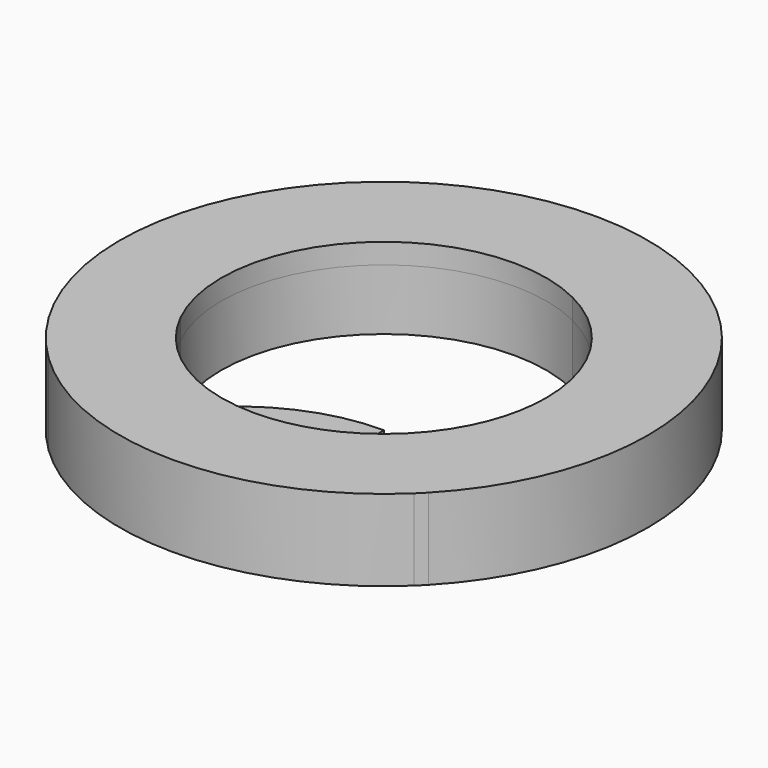
from build123d import *

# Parameters (mm, degrees)
F1_DEPTH = 20
F2_DEPTH = 15
F3_DEPTH = 15
F4_DEPTH = 5
F5_R     = 5


# Not quite as in the source:
# - a feature names something its author has since deleted; it is built from what else it names


with BuildPart() as f1:
    # F0 (on Top) → F1 (new body)
    with BuildSketch(Plane.XY):
        with BuildLine():
            ThreePointArc((-41.5739709642, -27.7777777778), (-35.3553390593, 35.3553390593), (27.7777777778, 41.5739709642))
            ThreePointArc((27.7777777778, 41.5739709642), (37.1759673359, 44.3146083461), (46.9444444444, 44.9579707705))
            ThreePointArc((46.9444444444, 44.9579707705), (-45.9619407771, 45.9619407771), (-44.9579707705, -46.9444444444))
            ThreePointArc((-44.9579707705, -46.9444444444), (-44.9806919732, -43.6819144147), (-44.7669675939, -40.426313036))
            ThreePointArc((-44.7669675939, -40.426313036), (-43.6312477339, -33.9857264796), (-41.5739709642, -27.7777777778))
        make_face()
        with BuildLine():
            ThreePointArc((45, -45), (36.220156419, -44.1351826403), (27.7777777778, -41.5739709642))
            ThreePointArc((27.7777777778, -41.5739709642), (14.5138115564, -47.8471448898), (0, -50))
            ThreePointArc((0, -50), (-12.7926961833, -48.3357727192), (-24.7337942073, -43.4538769745))
            ThreePointArc((-24.7337942073, -43.4538769745), (-29.4930498897, -42.6445374906), (-33.6593211472, -45.0833340912))
            ThreePointArc((-33.6593211472, -45.0833340912), (-40.9388886222, -46.870964929), (-44.7669675939, -40.426313036))
            ThreePointArc((-44.7669675939, -40.426313036), (-44.9806919732, -43.6819144147), (-44.9579707705, -46.9444444444))
            ThreePointArc((-44.9579707705, -46.9444444444), (0, -65), (44.9579707705, -46.9444444444))
            ThreePointArc((44.9579707705, -46.9444444444), (44.9894914656, -45.9724493115), (45, -45))
        make_face()
        with BuildLine():
            ThreePointArc((27.7777777778, 41.5739709642), (44.0958551844, 23.5702260396), (50, 0))
            ThreePointArc((50, 0), (47.8471448898, -14.5138115564), (41.5739709642, -27.7777777778))
            ThreePointArc((41.5739709642, -27.7777777778), (44.1351826403, -36.220156419), (45, -45))
            ThreePointArc((45, -45), (45.9724493115, -44.9894914656), (46.9444444444, -44.9579707705))
            ThreePointArc((46.9444444444, -44.9579707705), (60.317447264, -24.2240697562), (65, 0))
            ThreePointArc((65, 0), (60.317447264, 24.2240697562), (46.9444444444, 44.9579707705))
            ThreePointArc((46.9444444444, 44.9579707705), (37.1759673359, 44.3146083461), (27.7777777778, 41.5739709642))
        make_face()
        with BuildLine():
            ThreePointArc((45, -45), (44.1351826403, -36.220156419), (41.5739709642, -27.7777777778))
            ThreePointArc((41.5739709642, -27.7777777778), (35.3553390593, -35.3553390593), (27.7777777778, -41.5739709642))
            ThreePointArc((27.7777777778, -41.5739709642), (36.220156419, -44.1351826403), (45, -45))
        make_face()
        with BuildLine():
            ThreePointArc((46.9444444444, -44.9579707705), (45.9724493115, -44.9894914656), (45, -45))
            ThreePointArc((45, -45), (44.9894914656, -45.9724493115), (44.9579707705, -46.9444444444))
            ThreePointArc((44.9579707705, -46.9444444444), (45.9619407771, -45.9619407771), (46.9444444444, -44.9579707705))
        make_face()
        with BuildLine():
            ThreePointArc((-35.8322566591, -17.7777777778), (-28.2842712475, 28.2842712475), (17.7777777778, 35.8322566591))
            ThreePointArc((17.7777777778, 35.8322566591), (22.5931041578, 39.0247487976), (27.7777777778, 41.5739709642))
            ThreePointArc((27.7777777778, 41.5739709642), (-35.3553390593, 35.3553390593), (-41.5739709642, -27.7777777778))
            ThreePointArc((-41.5739709642, -27.7777777778), (-39.0247487976, -22.5931041578), (-35.8322566591, -17.7777777778))
        make_face()
        with BuildLine():
            ThreePointArc((17.7777777778, 35.8322566591), (33.993463424, 21.0818510678), (40, 0))
            Line((40, 0), (50, 0))
            ThreePointArc((50, 0), (44.0958551844, 23.5702260396), (27.7777777778, 41.5739709642))
            ThreePointArc((27.7777777778, 41.5739709642), (22.5931041578, 39.0247487976), (17.7777777778, 35.8322566591))
        make_face()
        with BuildLine():
            Line((50, 0), (40, 0))
            ThreePointArc((40, 0), (38.9441283531, -9.1298886531), (35.8322566591, -17.7777777778))
            ThreePointArc((35.8322566591, -17.7777777778), (39.0247487976, -22.5931041578), (41.5739709642, -27.7777777778))
            ThreePointArc((41.5739709642, -27.7777777778), (47.8471448898, -14.5138115564), (50, 0))
        make_face()
        with BuildLine():
            ThreePointArc((41.5739709642, -27.7777777778), (39.0247487976, -22.5931041578), (35.8322566591, -17.7777777778))
            ThreePointArc((35.8322566591, -17.7777777778), (28.2842712475, -28.2842712475), (17.7777777778, -35.8322566591))
            ThreePointArc((17.7777777778, -35.8322566591), (22.5931041578, -39.0247487976), (27.7777777778, -41.5739709642))
            ThreePointArc((27.7777777778, -41.5739709642), (35.3553390593, -35.3553390593), (41.5739709642, -27.7777777778))
        make_face()
        with BuildLine():
            ThreePointArc((27.7777777778, -41.5739709642), (22.5931041578, -39.0247487976), (17.7777777778, -35.8322566591))
            ThreePointArc((17.7777777778, -35.8322566591), (9.1298886531, -38.9441283531), (0, -40))
            Line((0, -40), (0, -50))
            ThreePointArc((0, -50), (14.5138115564, -47.8471448898), (27.7777777778, -41.5739709642))
        make_face()
        with BuildLine():
            ThreePointArc((0, -40), (-21.0818510678, -33.993463424), (-35.8322566591, -17.7777777778))
            ThreePointArc((-35.8322566591, -17.7777777778), (-39.0247487976, -22.5931041578), (-41.5739709642, -27.7777777778))
            ThreePointArc((-41.5739709642, -27.7777777778), (-38.1355654332, -32.3369548518), (-34.1997389873, -36.4743451373))
            ThreePointArc((-34.1997389873, -36.4743451373), (-29.6726945164, -40.2433994605), (-24.7337942073, -43.4538769745))
            ThreePointArc((-24.7337942073, -43.4538769745), (-12.7926961833, -48.3357727192), (0, -50))
            Line((0, -50), (0, -40))
        make_face()
        with BuildLine():
            ThreePointArc((-34.1997389873, -36.4743451373), (-38.1355654332, -32.3369548518), (-41.5739709642, -27.7777777778))
            ThreePointArc((-41.5739709642, -27.7777777778), (-43.6312477339, -33.9857264796), (-44.7669675939, -40.426313036))
            ThreePointArc((-44.7669675939, -40.426313036), (-40.7099854287, -35.1704182799), (-34.1997389873, -36.4743451373))
        make_face()
        with BuildLine():
            ThreePointArc((-32.2106591377, -41.0660656442), (-32.729295856, -38.564049664), (-34.1997389873, -36.4743451373))
            ThreePointArc((-34.1997389873, -36.4743451373), (-40.7099854287, -35.1704182799), (-44.7669675939, -40.426313036))
            ThreePointArc((-44.7669675939, -40.426313036), (-40.9388886222, -46.870964929), (-33.6593211472, -45.0833340912))
            ThreePointArc((-33.6593211472, -45.0833340912), (-32.5838900439, -43.2013096228), (-32.2106591377, -41.0660656442))
        make_face()
        with BuildLine():
            ThreePointArc((-24.7337942073, -43.4538769745), (-29.6726945164, -40.2433994605), (-34.1997389873, -36.4743451373))
            ThreePointArc((-34.1997389873, -36.4743451373), (-32.729295856, -38.564049664), (-32.2106591377, -41.0660656442))
            ThreePointArc((-32.2106591377, -41.0660656442), (-32.5838900439, -43.2013096228), (-33.6593211472, -45.0833340912))
            ThreePointArc((-33.6593211472, -45.0833340912), (-29.4930498897, -42.6445374906), (-24.7337942073, -43.4538769745))
        make_face()
    extrude(amount=F1_DEPTH)

    # F0 (on Top) → F2 (cut)
    with BuildSketch(Plane.XY):
        with BuildLine():
            ThreePointArc((17.7777777778, 35.8322566591), (33.993463424, 21.0818510678), (40, 0))
            Line((40, 0), (50, 0))
            ThreePointArc((50, 0), (44.0958551844, 23.5702260396), (27.7777777778, 41.5739709642))
            ThreePointArc((27.7777777778, 41.5739709642), (22.5931041578, 39.0247487976), (17.7777777778, 35.8322566591))
        make_face()
        with BuildLine():
            Line((50, 0), (40, 0))
            ThreePointArc((40, 0), (38.9441283531, -9.1298886531), (35.8322566591, -17.7777777778))
            ThreePointArc((35.8322566591, -17.7777777778), (39.0247487976, -22.5931041578), (41.5739709642, -27.7777777778))
            ThreePointArc((41.5739709642, -27.7777777778), (47.8471448898, -14.5138115564), (50, 0))
        make_face()
        with BuildLine():
            ThreePointArc((41.5739709642, -27.7777777778), (39.0247487976, -22.5931041578), (35.8322566591, -17.7777777778))
            ThreePointArc((35.8322566591, -17.7777777778), (28.2842712475, -28.2842712475), (17.7777777778, -35.8322566591))
            ThreePointArc((17.7777777778, -35.8322566591), (22.5931041578, -39.0247487976), (27.7777777778, -41.5739709642))
            ThreePointArc((27.7777777778, -41.5739709642), (35.3553390593, -35.3553390593), (41.5739709642, -27.7777777778))
        make_face()
        with BuildLine():
            ThreePointArc((27.7777777778, -41.5739709642), (22.5931041578, -39.0247487976), (17.7777777778, -35.8322566591))
            ThreePointArc((17.7777777778, -35.8322566591), (9.1298886531, -38.9441283531), (0, -40))
            Line((0, -40), (0, -50))
            ThreePointArc((0, -50), (14.5138115564, -47.8471448898), (27.7777777778, -41.5739709642))
        make_face()
        with BuildLine():
            ThreePointArc((0, -40), (-21.0818510678, -33.993463424), (-35.8322566591, -17.7777777778))
            ThreePointArc((-35.8322566591, -17.7777777778), (-39.0247487976, -22.5931041578), (-41.5739709642, -27.7777777778))
            ThreePointArc((-41.5739709642, -27.7777777778), (-38.1355654332, -32.3369548518), (-34.1997389873, -36.4743451373))
            ThreePointArc((-34.1997389873, -36.4743451373), (-29.6726945164, -40.2433994605), (-24.7337942073, -43.4538769745))
            ThreePointArc((-24.7337942073, -43.4538769745), (-12.7926961833, -48.3357727192), (0, -50))
            Line((0, -50), (0, -40))
        make_face()
        with BuildLine():
            ThreePointArc((-35.8322566591, -17.7777777778), (-28.2842712475, 28.2842712475), (17.7777777778, 35.8322566591))
            ThreePointArc((17.7777777778, 35.8322566591), (22.5931041578, 39.0247487976), (27.7777777778, 41.5739709642))
            ThreePointArc((27.7777777778, 41.5739709642), (-35.3553390593, 35.3553390593), (-41.5739709642, -27.7777777778))
            ThreePointArc((-41.5739709642, -27.7777777778), (-39.0247487976, -22.5931041578), (-35.8322566591, -17.7777777778))
        make_face()
    extrude(amount=F2_DEPTH, mode=Mode.SUBTRACT)


with BuildPart() as f3:
    # F0 (on Top) → F3 (new body)
    with BuildSketch(Plane.XY):
        with BuildLine():
            ThreePointArc((0, -40), (-21.0818510678, -33.993463424), (-35.8322566591, -17.7777777778))
            ThreePointArc((-35.8322566591, -17.7777777778), (-39.0247487976, -22.5931041578), (-41.5739709642, -27.7777777778))
            ThreePointArc((-41.5739709642, -27.7777777778), (-38.1355654332, -32.3369548518), (-34.1997389873, -36.4743451373))
            ThreePointArc((-34.1997389873, -36.4743451373), (-29.6726945164, -40.2433994605), (-24.7337942073, -43.4538769745))
            ThreePointArc((-24.7337942073, -43.4538769745), (-12.7926961833, -48.3357727192), (0, -50))
            Line((0, -50), (0, -40))
        make_face()
        with BuildLine():
            ThreePointArc((27.7777777778, -41.5739709642), (22.5931041578, -39.0247487976), (17.7777777778, -35.8322566591))
            ThreePointArc((17.7777777778, -35.8322566591), (9.1298886531, -38.9441283531), (0, -40))
            Line((0, -40), (0, -50))
            ThreePointArc((0, -50), (14.5138115564, -47.8471448898), (27.7777777778, -41.5739709642))
        make_face()
        with BuildLine():
            ThreePointArc((41.5739709642, -27.7777777778), (39.0247487976, -22.5931041578), (35.8322566591, -17.7777777778))
            ThreePointArc((35.8322566591, -17.7777777778), (28.2842712475, -28.2842712475), (17.7777777778, -35.8322566591))
            ThreePointArc((17.7777777778, -35.8322566591), (22.5931041578, -39.0247487976), (27.7777777778, -41.5739709642))
            ThreePointArc((27.7777777778, -41.5739709642), (35.3553390593, -35.3553390593), (41.5739709642, -27.7777777778))
        make_face()
        with BuildLine():
            Line((50, 0), (40, 0))
            ThreePointArc((40, 0), (38.9441283531, -9.1298886531), (35.8322566591, -17.7777777778))
            ThreePointArc((35.8322566591, -17.7777777778), (39.0247487976, -22.5931041578), (41.5739709642, -27.7777777778))
            ThreePointArc((41.5739709642, -27.7777777778), (47.8471448898, -14.5138115564), (50, 0))
        make_face()
        with BuildLine():
            ThreePointArc((17.7777777778, 35.8322566591), (33.993463424, 21.0818510678), (40, 0))
            Line((40, 0), (50, 0))
            ThreePointArc((50, 0), (44.0958551844, 23.5702260396), (27.7777777778, 41.5739709642))
            ThreePointArc((27.7777777778, 41.5739709642), (22.5931041578, 39.0247487976), (17.7777777778, 35.8322566591))
        make_face()
        with BuildLine():
            ThreePointArc((-35.8322566591, -17.7777777778), (-28.2842712475, 28.2842712475), (17.7777777778, 35.8322566591))
            ThreePointArc((17.7777777778, 35.8322566591), (22.5931041578, 39.0247487976), (27.7777777778, 41.5739709642))
            ThreePointArc((27.7777777778, 41.5739709642), (-35.3553390593, 35.3553390593), (-41.5739709642, -27.7777777778))
            ThreePointArc((-41.5739709642, -27.7777777778), (-39.0247487976, -22.5931041578), (-35.8322566591, -17.7777777778))
        make_face()
    extrude(amount=F3_DEPTH)


with BuildPart() as f4:
    # F0 (on Top) → F4 (new body)
    with BuildSketch(Plane.XY):
        with BuildLine():
            ThreePointArc((0, 0), (-20, -4.6887112585), (-35.8322566591, -17.7777777778))
            ThreePointArc((-35.8322566591, -17.7777777778), (-21.0818510678, -33.993463424), (0, -40))
            ThreePointArc((0, -40), (9.1298886531, -38.9441283531), (17.7777777778, -35.8322566591))
            ThreePointArc((17.7777777778, -35.8322566591), (4.6887112585, -20), (0, 0))
        make_face()
        with BuildLine():
            ThreePointArc((27.7777777778, -41.5739709642), (22.5931041578, -39.0247487976), (17.7777777778, -35.8322566591))
            ThreePointArc((17.7777777778, -35.8322566591), (9.1298886531, -38.9441283531), (0, -40))
            Line((0, -40), (0, -50))
            ThreePointArc((0, -50), (14.5138115564, -47.8471448898), (27.7777777778, -41.5739709642))
        make_face()
        with BuildLine():
            ThreePointArc((0, -40), (-21.0818510678, -33.993463424), (-35.8322566591, -17.7777777778))
            ThreePointArc((-35.8322566591, -17.7777777778), (-39.0247487976, -22.5931041578), (-41.5739709642, -27.7777777778))
            ThreePointArc((-41.5739709642, -27.7777777778), (-38.1355654332, -32.3369548518), (-34.1997389873, -36.4743451373))
            ThreePointArc((-34.1997389873, -36.4743451373), (-29.6726945164, -40.2433994605), (-24.7337942073, -43.4538769745))
            ThreePointArc((-24.7337942073, -43.4538769745), (-12.7926961833, -48.3357727192), (0, -50))
            Line((0, -50), (0, -40))
        make_face()
        with BuildLine():
            ThreePointArc((-34.1997389873, -36.4743451373), (-38.1355654332, -32.3369548518), (-41.5739709642, -27.7777777778))
            ThreePointArc((-41.5739709642, -27.7777777778), (-43.6312477339, -33.9857264796), (-44.7669675939, -40.426313036))
            ThreePointArc((-44.7669675939, -40.426313036), (-40.7099854287, -35.1704182799), (-34.1997389873, -36.4743451373))
        make_face()
        with BuildLine():
            ThreePointArc((-32.2106591377, -41.0660656442), (-32.729295856, -38.564049664), (-34.1997389873, -36.4743451373))
            ThreePointArc((-34.1997389873, -36.4743451373), (-40.7099854287, -35.1704182799), (-44.7669675939, -40.426313036))
            ThreePointArc((-44.7669675939, -40.426313036), (-40.9388886222, -46.870964929), (-33.6593211472, -45.0833340912))
            ThreePointArc((-33.6593211472, -45.0833340912), (-32.5838900439, -43.2013096228), (-32.2106591377, -41.0660656442))
        make_face()
        with BuildLine():
            ThreePointArc((-24.7337942073, -43.4538769745), (-29.6726945164, -40.2433994605), (-34.1997389873, -36.4743451373))
            ThreePointArc((-34.1997389873, -36.4743451373), (-32.729295856, -38.564049664), (-32.2106591377, -41.0660656442))
            ThreePointArc((-32.2106591377, -41.0660656442), (-32.5838900439, -43.2013096228), (-33.6593211472, -45.0833340912))
            ThreePointArc((-33.6593211472, -45.0833340912), (-29.4930498897, -42.6445374906), (-24.7337942073, -43.4538769745))
        make_face()
    extrude(amount=-F4_DEPTH)

    # F5
    f5_edges = [f4.edges().sort_by_distance(p)[0] for p in [
        (27.777778, -41.573971, -2.5),
    ]]
    fillet(f5_edges, radius=F5_R)


solid = Compound([f1.part, f3.part, f4.part])
